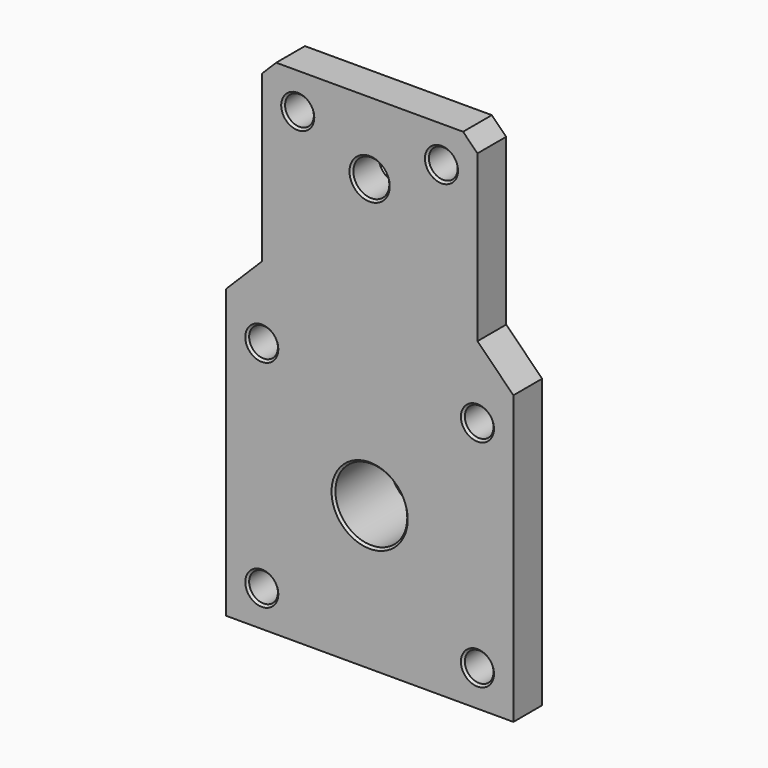
from build123d import *

# Parameters (mm, degrees)
F0_R     = 19.05
F1_DEPTH = 6.35
F2_R     = 3.175
F3_DEPTH = 6.35
F4_SIZE  = 0.762
F5_R     = 6.35
F5_R_2   = 2.54
F6_DEPTH = 12.7
F7_SIZE  = 0.381
F8_SIZE  = 6.34999
F9_SIZE  = 2.54


# Not quite as in the source:
# - a fillet or chamfer is up to 0.001 mm smaller than in the source, because OpenCascade refuses the exact size


with BuildPart() as f1:
    # F0 (on Front) → F1 (new body)
    with BuildSketch(Plane.XZ):
        Circle(F0_R)
    extrude(amount=F1_DEPTH)

    # F2 (on face) → F3 (join)
    with BuildSketch(Plane.XZ.offset(6.35)):
        Polygon((-19.05, 25.4), (-25.4, 25.4), (-25.4, -25.4), (25.4, -25.4), (25.4, 25.4), (19.05, 25.4), (19.05, 63.5), (-19.05, 63.5), align=None)
        with Locations((0, 50.8)):
            Circle(F2_R, mode=Mode.SUBTRACT)
    extrude(amount=F3_DEPTH)

    # F4
    f4_edges = [f1.edges().sort_by_distance(p)[0] for p in [
        (-19.05, 0, 0),
    ]]
    chamfer(f4_edges, length=F4_SIZE)

    # F5 (on face) → F6 (cut)
    with BuildSketch(Plane.XZ.offset(12.7)):
        Circle(F5_R)
        with Locations((-19.05, 19.05)):
            Circle(F5_R_2)
        with Locations((19.05, 19.05)):
            Circle(F5_R_2)
        with Locations((19.05, -19.05)):
            Circle(F5_R_2)
        with Locations((-19.05, -19.05)):
            Circle(F5_R_2)
        with Locations((-12.7, 57.15)):
            Circle(F5_R_2)
        with Locations((12.7, 57.15)):
            Circle(F5_R_2)
    extrude(amount=-F6_DEPTH, mode=Mode.SUBTRACT)

    # F7
    f7_edges = [f1.edges().sort_by_distance(p)[0] for p in [
        (-21.59, -12.7, 19.05),
        (16.51, -12.7, 19.05),
        (16.51, -12.7, -19.05),
        (-21.59, -12.7, -19.05),
        (-6.35, -12.7, 0),
        (-6.35, 0, 0),
        (16.51, -6.35, -19.05),
        (-21.59, -6.35, -19.05),
        (-21.59, -6.35, 19.05),
        (16.51, -6.35, 19.05),
        (-15.24, -12.7, 57.15),
        (10.16, -12.7, 57.15),
        (-15.24, -6.35, 57.15),
        (10.16, -6.35, 57.15),
        (-3.175, -6.35, 50.8),
        (-3.175, -12.7, 50.8),
    ]]
    chamfer(f7_edges, length=F7_SIZE)

    # F8 (size 6.35 in the source; OpenCascade refuses exactly that, so slightly less here)
    f8_edges = [f1.edges().sort_by_distance(p)[0] for p in [
        (-19.05, -9.525, 25.4),
        (19.05, -9.525, 25.4),
    ]]
    chamfer(f8_edges, length=F8_SIZE)

    # F9
    f9_edges = [f1.edges().sort_by_distance(p)[0] for p in [
        (-19.05, -9.525, 63.5),
        (19.05, -9.525, 63.5),
    ]]
    chamfer(f9_edges, length=F9_SIZE)


solid = f1.part
